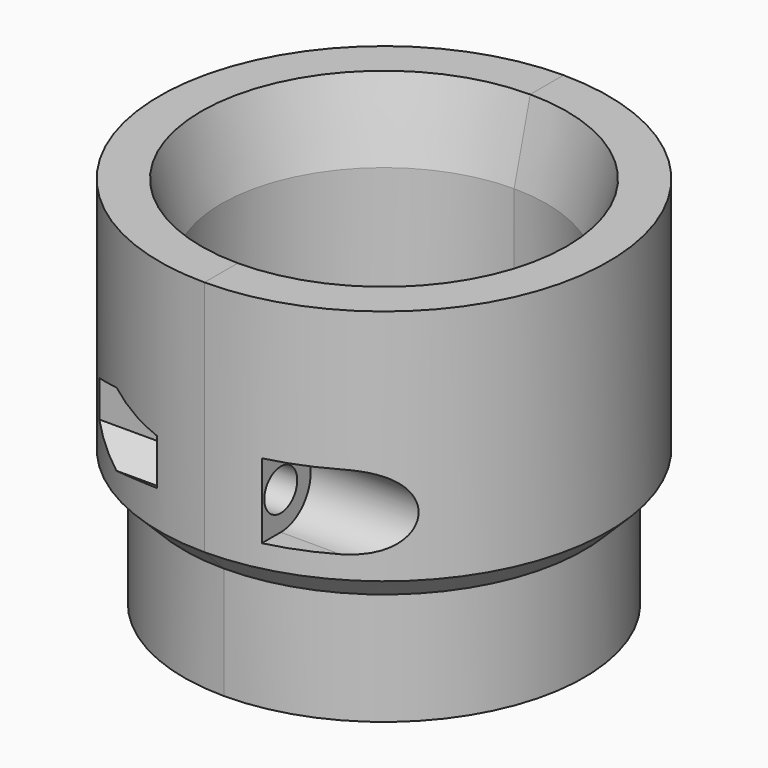
from build123d import *

# Parameters (mm, degrees)
F1_ANGLE  = 180
F5_DEPTH  = 82.4
F7_D      = 5.5
F7_2_D    = 5.5
F10_DEPTH = 30


# Not quite as in the source:
# - a pattern or mirror of a feature is missing from the dataset's text; its kind, count and spacing are read off the source's solid


with BuildPart() as f1:
    # F0 (on Right) → F1 (revolve)
    with BuildSketch(Plane.YZ):
        Polygon((-30, 18.25), (-26.75, 15), (-26.75, 0), (-24, 0), (-21.75, 6.1818241938), (-21.75, 40), (-24.4294919243, 50), (-30, 50), align=None)
    revolve(axis=Axis((0, 0, 27.1151401103), (0, 0, 1)), revolution_arc=F1_ANGLE)


with BuildPart() as f3_1:
    # F3: instance of F1
    add(f1.part.mirror(Plane.YZ))

    # F7#2 (through all)
    with Locations(Plane.YZ.offset(7)):
        with Locations((-26, 26.25)):
            f7_2 = Hole(F7_2_D / 2)

    # F7_2_copies: F7#2 across plane
    add(f7_2.mirror(Plane.ZX), mode=Mode.SUBTRACT)

    # F9 (on offset) → F10 (cut)
    with BuildSketch(Plane.YZ.offset(-7)):
        Polygon((-21.75, 28.7037386441), (-26, 31.1574772881), (-30.25, 28.7037386441), (-30.25, 23.7962613559), (-26, 21.3425227119), (-21.75, 23.7962613559), align=None)
        Polygon((21.75, 28.7037386441), (21.75, 23.7962613559), (26, 21.3425227119), (30.25, 23.7962613559), (30.25, 28.7037386441), (26, 31.1574772881), align=None)
    extrude(amount=-F10_DEPTH, mode=Mode.SUBTRACT)


with BuildPart() as f1_1:
    add(f1.part)

    # F4 (on offset) → F5 (cut)
    with BuildSketch(Plane.YZ.offset(7)):
        with BuildLine():
            ThreePointArc((-26, 21.25), (-21, 26.25), (-26, 31.25))
            Line((-26, 31.25), (-30, 31.25))
            Line((-30, 31.25), (-30, 21.25))
            Line((-30, 21.25), (-26, 21.25))
        make_face()
    f5 = extrude(amount=F5_DEPTH, mode=Mode.SUBTRACT)

    # F5_copies: F5 across plane
    add(f5.mirror(Plane(origin=(0, -2.4e-05, 0), x_dir=(1, 1e-06, 0), z_dir=(-1e-06, 1, 0))), mode=Mode.SUBTRACT)

    # F7 (through all)
    with Locations(Plane.YZ.offset(7)):
        with Locations((-26, 26.25)):
            f7 = Hole(F7_D / 2)

    # F7_copies: F7 across plane
    add(f7.mirror(Plane.ZX), mode=Mode.SUBTRACT)


solid = Compound([f3_1.part, f1_1.part])
